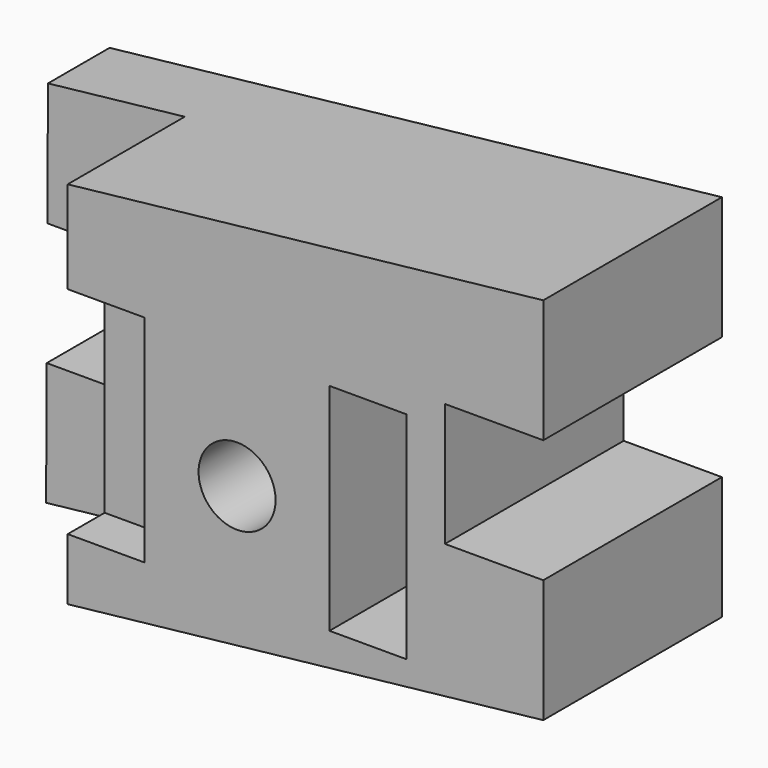
from build123d import *

# Parameters (mm, degrees)
F0_R     = 15.875
F1_DEPTH = 31.75
F2_DEPTH = 92.075
F0_W     = 31.75
F0_H     = 88.9
F3_DEPTH = 73.025
F4_DEPTH = 53.975


# Not quite as in the source:
# - a feature names something its author has since deleted; it is built from what else it names


with BuildPart() as f1:
    # F0 (on Front) → F1 (new body)
    with BuildSketch(Plane.XZ):
        Polygon((-69.8361151936, 86.826035718), (-126.218325014, 80.5985571647), (-126.4791783958, 29.7122203269), (-85.725, 29.7122203269), (-85.725, -21.0877796731), (-126.7395891979, -21.0877796731), (-127, -71.8877796731), (-69.8361151936, -65.5739758634), (-69.8361151936, -40.1377796731), (-69.8361151936, 48.7622203269), align=None)
        Polygon((126.2463778257, 108.4835678339), (-69.8361151936, 86.826035718), (-69.8361151936, 48.7622203269), (-38.0861151936, 48.7622203269), (-38.0861151936, -40.1377796731), (-38.0861151936, -62.0671590745), (38.1138848064, -53.6507987812), (38.1138848064, -40.1378311361), (38.1138848064, 48.7622203269), (69.8638848064, 48.7622203269), (69.8638848064, -40.1378311361), (69.8638848064, -50.1439819923), (126.2463778257, -43.9164836263), (126.2463778257, 6.8835678339), (85.725, 6.8835678339), (85.725, 57.6835678339), (126.2463778257, 57.6835678339), align=None)
        Circle(F0_R, mode=Mode.SUBTRACT)
        Polygon((-38.0861151936, -40.1377796731), (-69.8361151936, -40.1377796731), (-69.8361151936, -65.5739758634), (-38.0861151936, -62.0671590745), align=None)
    extrude(amount=F1_DEPTH)

    # F0 (on Front) → F2 (join)
    with BuildSketch(Plane.XZ):
        Polygon((126.2463778257, 108.4835678339), (-69.8361151936, 86.826035718), (-69.8361151936, 48.7622203269), (-38.0861151936, 48.7622203269), (-38.0861151936, -40.1377796731), (-38.0861151936, -62.0671590745), (38.1138848064, -53.6507987812), (38.1138848064, -40.1378311361), (38.1138848064, 48.7622203269), (69.8638848064, 48.7622203269), (69.8638848064, -40.1378311361), (69.8638848064, -50.1439819923), (126.2463778257, -43.9164836263), (126.2463778257, 6.8835678339), (85.725, 6.8835678339), (85.725, 57.6835678339), (126.2463778257, 57.6835678339), align=None)
        Circle(F0_R, mode=Mode.SUBTRACT)
        Polygon((-38.0861151936, -40.1377796731), (-69.8361151936, -40.1377796731), (-69.8361151936, -65.5739758634), (-38.0861151936, -62.0671590745), align=None)
        Polygon((38.1138848064, -40.1378311361), (38.1138848064, -53.6507987812), (69.8638848064, -50.1439819923), (69.8638848064, -40.1378311361), align=None)
    extrude(amount=F2_DEPTH)

    # F0 (on Front) → F3 (join)
    with BuildSketch(Plane.XZ):
        with Locations((-53.9611151936, 4.3122203269)):
            Rectangle(F0_W, F0_H)
    extrude(amount=F3_DEPTH)

    # F0 (on Front) → F4 (join)
    with BuildSketch(Plane.XZ):
        Polygon((126.2463778257, 108.4835678339), (-69.8361151936, 86.826035718), (-69.8361151936, 48.7622203269), (-38.0861151936, 48.7622203269), (-38.0861151936, -40.1377796731), (-38.0861151936, -62.0671590745), (38.1138848064, -53.6507987812), (38.1138848064, -40.1378311361), (38.1138848064, 48.7622203269), (69.8638848064, 48.7622203269), (69.8638848064, -40.1378311361), (69.8638848064, -50.1439819923), (126.2463778257, -43.9164836263), (126.2463778257, 6.8835678339), (85.725, 6.8835678339), (85.725, 57.6835678339), (126.2463778257, 57.6835678339), align=None)
        Circle(F0_R, mode=Mode.SUBTRACT)
    extrude(amount=F4_DEPTH)


solid = f1.part
